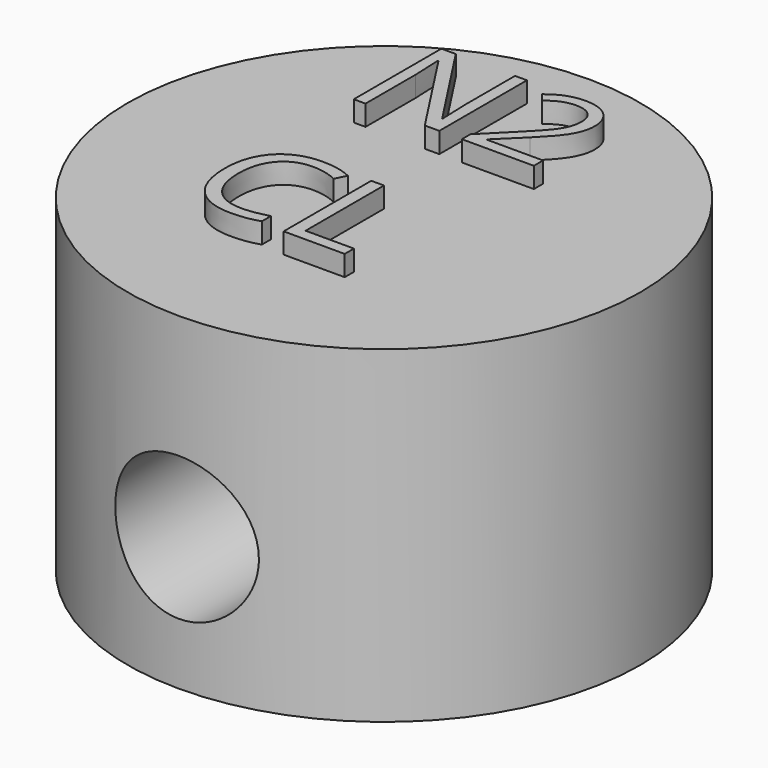
from build123d import *

# Parameters (mm, degrees)
F0_R         = 12.5
F1_DEPTH     = 16
F3_R         = 3.5
F4_DEPTH     = 25.001
F5_TEXT_SIZE = 7.4801309023
F6_DEPTH     = 1


# Not quite as in the source:
# - Text() gives the source's letters only with a copy of the font that has no kerning and outlines rounded to 1/6400 em; it was checked with that copy


with BuildPart() as f1:
    # F0 (on Top) → F1 (new body)
    with BuildSketch(Plane.XY):
        Circle(F0_R)
    extrude(amount=F1_DEPTH)

    # F3 (on offset) → F4 (cut, through all)
    with BuildSketch(Plane.XZ.offset(-12.5)):
        with Locations((0, 6.5)):
            Circle(F3_R)
    extrude(amount=F4_DEPTH, mode=Mode.SUBTRACT)

    # F5 (on face) → F6 (join)
    with BuildSketch(Plane.XY.offset(16)):
        with Locations((-5.5, 4.1143057504)):
            Text('N2', F5_TEXT_SIZE, font='Open Sans', text_align=(TextAlign.LEFT, TextAlign.BOTTOM))
        with Locations((-5.5, -6.0586722768)):
            Text('CL', F5_TEXT_SIZE, font='Open Sans', text_align=(TextAlign.LEFT, TextAlign.BOTTOM))
    extrude(amount=F6_DEPTH)


solid = f1.part
